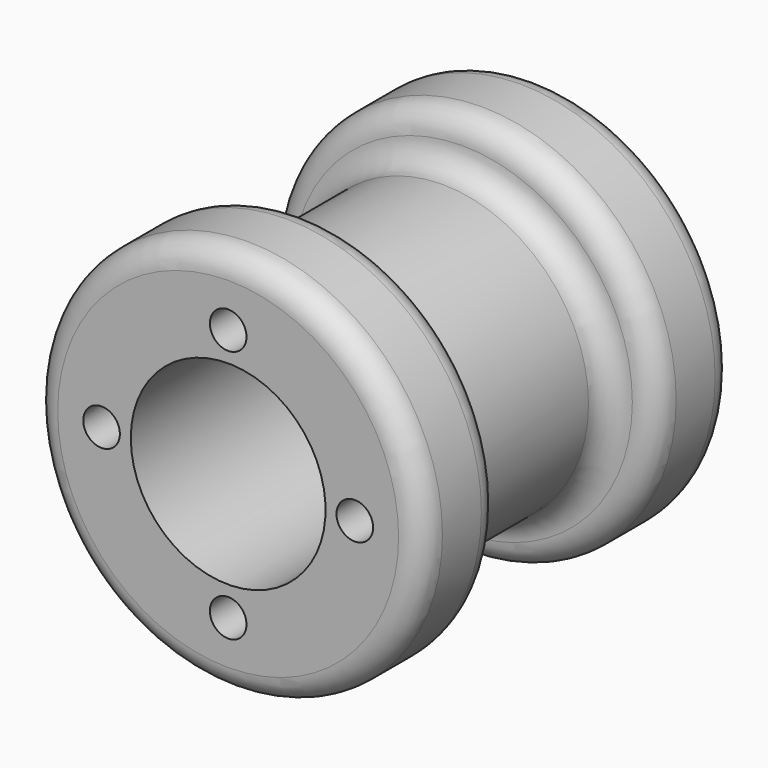
from build123d import *

# Parameters (mm, degrees)
F0_R     = 12.7
F1_DEPTH = 6.35
F2_R     = 9.525
F3_DEPTH = 12.7
F4_R     = 12.7
F5_DEPTH = 6.35
F7_D     = 12.7
F8_D     = 2.3876
F8_DEPTH = 3.175
F8_TIP   = 0.717307407
F9_R     = 1.58749


# Not quite as in the source:
# - a fillet or chamfer is up to 0.001 mm smaller than in the source, because OpenCascade refuses the exact size


with BuildPart() as f1:
    # F0 (on Front) → F1 (new body)
    with BuildSketch(Plane.XZ):
        Circle(F0_R)
    extrude(amount=F1_DEPTH)

    # F2 (on face) → F3 (join)
    with BuildSketch(Plane.XZ.offset(6.35)):
        Circle(F2_R)
    extrude(amount=F3_DEPTH)

    # F4 (on face) → F5 (join)
    with BuildSketch(Plane.XZ.offset(19.05)):
        Circle(F4_R)
    extrude(amount=F5_DEPTH)

    # F7 (through all)
    with Locations(Plane.XZ.offset(25.4)):
        with Locations((0, 0)):
            Hole(F7_D / 2)

    # F8
    with Locations(Plane.XZ.offset(25.4)):
        with Locations((-8.255, 0), (0, 8.255), (8.255, 0), (0, -8.255)):
            Hole(F8_D / 2, depth=F8_DEPTH)
            with Locations((0, 0, -(F8_DEPTH + F8_TIP / 2))):  # 118° drill point
                Cone(0, F8_D / 2, F8_TIP, mode=Mode.SUBTRACT)

    # F9 (radius 1.5875 in the source; OpenCascade refuses exactly that, so slightly less here)
    f9_edges = [f1.edges().sort_by_distance(p)[0] for p in [
        (-12.7, -25.4, 0),
        (-12.7, -19.05, 0),
        (-12.7, -6.35, 0),
        (-12.7, 0, 0),
        (-9.525, -6.35, 0),
        (-9.525, -19.05, 0),
    ]]
    fillet(f9_edges, radius=F9_R)


solid = f1.part
